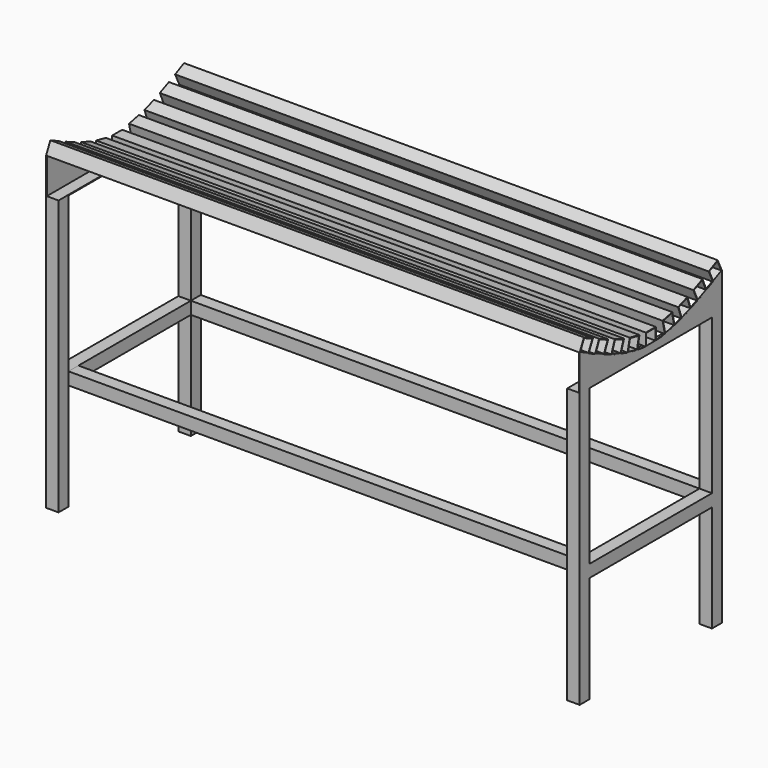
from build123d import *

# Parameters (mm, degrees)
F1_DEPTH  = 2
F2_W      = 35
F2_H      = 500
F3_DEPTH  = 2
F6_W      = 35
F6_H      = 35
F6_W_2    = 32
F6_H_2    = 32
F7_DEPTH  = 1500
F9_DEPTH  = 1500
F11_DEPTH = 1500
F13_DEPTH = 1500
F14_W     = 35
F14_H     = 35
F14_W_2   = 33
F14_H_2   = 33
F15_DEPTH = 770
F16_W     = 35
F16_H     = 35
F16_W_2   = 33
F16_H_2   = 33
F17_DEPTH = 770
F18_W     = 35
F18_H     = 35
F18_W_2   = 33
F18_H_2   = 33
F19_DEPTH = 440
F20_W     = 35
F20_H     = 35
F20_W_2   = 33
F20_H_2   = 33
F21_DEPTH = 440
F22_W     = 35
F22_H     = 35
F22_W_2   = 33
F22_H_2   = 33
F23_DEPTH = 1430
F24_W     = 35
F24_H     = 35
F24_W_2   = 33
F24_H_2   = 33
F25_DEPTH = 1430


with BuildPart() as f1:
    # F0 (on Right) → F1 (new body)
    with BuildSketch(Plane.YZ):
        with BuildLine():
            Line((-250, 50), (-250, -50))
            Line((-250, -50), (250, -50))
            Line((250, -50), (250, 50))
            add(Edge.make_bspline(
                [(250, 50), (166.6666666667, 10), (0, -70), (-166.6666666667, 10), (-250, 50)],
                knots=[0, 0, 0, 0, 0.5, 1, 1, 1, 1], degree=3))
        make_face()
    extrude(amount=F1_DEPTH)

    # F2 (on face) → F3 (join)
    with BuildSketch(Plane(origin=(0, 0, -50), x_dir=(1, 0, 0), z_dir=(0, 0, -1))):
        with Locations((17.5, 0)):
            Rectangle(F2_W, F2_H)
    extrude(amount=F3_DEPTH)


with BuildPart() as f4_1:
    # F4: instance of F1
    add(f1.part.mirror(Plane(origin=(35, 0, -51), x_dir=(0, 1, 0), z_dir=(1, 0, 0))))


with BuildPart() as f4_1_1:
    # F5: moved
    add(f4_1.part.moved(Location((1430, 0, 0))))

    # F16 (on face) → F17 (join)
    with BuildSketch(Plane(origin=(0, 0, -52), x_dir=(1, 0, 0), z_dir=(0, 0, -1))):
        with Locations((1482.5, 232.5)):
            Rectangle(F16_W, F16_H)
        with Locations((1482.5, 232.5)):
            Rectangle(F16_W_2, F16_H_2, mode=Mode.SUBTRACT)
        with Locations((1482.5, -232.5)):
            Rectangle(F16_W, F16_H)
        with Locations((1482.5, -232.5)):
            Rectangle(F16_W_2, F16_H_2, mode=Mode.SUBTRACT)
    extrude(amount=F17_DEPTH)

    # F18 (on face) → F19 (join)
    with BuildSketch(Plane.XZ.offset(-215)):
        with Locations((1482.5, -504.5)):
            Rectangle(F18_W, F18_H)
        with Locations((1482.5, -504.5)):
            Rectangle(F18_W_2, F18_H_2, mode=Mode.SUBTRACT)
    extrude(amount=F19_DEPTH)


with BuildPart() as f1_1:
    add(f1.part)

    # F6 (on face) → F7 (join)
    with BuildSketch(Plane(origin=(0, 0, 0), x_dir=(0, -1, 0), z_dir=(-1, 0, 0))):
        with Locations((0, -12.5)):
            Rectangle(F6_W, F6_H)
        with Locations((0, -12.5)):
            Rectangle(F6_W_2, F6_H_2, mode=Mode.SUBTRACT)
    extrude(amount=-F7_DEPTH)

    # F14 (on face) → F15 (join)
    with BuildSketch(Plane(origin=(0, 0, -52), x_dir=(1, 0, 0), z_dir=(0, 0, -1))):
        with Locations((17.5, 232.5)):
            Rectangle(F14_W, F14_H)
        with Locations((17.5, 232.5)):
            Rectangle(F14_W_2, F14_H_2, mode=Mode.SUBTRACT)
        with Locations((17.5, -232.5)):
            Rectangle(F14_W, F14_H)
        with Locations((17.5, -232.5)):
            Rectangle(F14_W_2, F14_H_2, mode=Mode.SUBTRACT)
    extrude(amount=F15_DEPTH)

    # F20 (on face) → F21 (join)
    with BuildSketch(Plane.XZ.offset(-215)):
        with Locations((17.5, -504.5)):
            Rectangle(F20_W, F20_H)
        with Locations((17.5, -504.5)):
            Rectangle(F20_W_2, F20_H_2, mode=Mode.SUBTRACT)
    extrude(amount=F21_DEPTH)


with BuildPart() as f9:
    # F8 (on face) → F9 (new body)
    with BuildSketch(Plane(origin=(0, 0, 0), x_dir=(0, -1, 0), z_dir=(-1, 0, 0))):
        Polygon((-234.9200030965, 81.5847066377), (-250, 50), (-218.4152933623, 34.9200030965), (-203.3352964588, 66.5047097342), align=None)
        Polygon((-234.2126583936, 79.5847907717), (-219.7739353592, 72.6910779015), (-205.3352123248, 65.7973650313), (-219.1226380652, 36.9199189626), (-248.0000841339, 50.7073447029), align=None, mode=Mode.SUBTRACT)
    extrude(amount=-F9_DEPTH)


with BuildPart() as f11:
    # F10 (on face) → F11 (new body)
    with BuildSketch(Plane(origin=(0, 0, 0), x_dir=(0, -1, 0), z_dir=(-1, 0, 0))):
        with BuildLine():
            add(Edge.make_bspline(
                [(-83.6444792813, -18.0650520534), (-72.2522280284, -21.1120515617), (-60.8599767755, -23.6616132493), (-49.4677255225, -25.6115414701)],
                knots=[0.3327110414, 0.3327110414, 0.3327110414, 0.3327110414, 0.401064549, 0.401064549, 0.401064549, 0.401064549], degree=3))
            Line((-49.4677255225, -25.6115414701), (-41.5525741961, 10.2348187258))
            Line((-41.5525741961, 10.2348187258), (-75.7293279548, 17.7813081425))
            Line((-75.7293279548, 17.7813081425), (-83.6444792813, -18.0650520534))
        make_face()
        Polygon((-74.6562526953, 16.0082330425), (-58.9643720505, 12.5433454159), (-43.2724914057, 9.0784577893), (-50.5408007821, -23.8384663701), (-81.9245620717, -16.9086911169), align=None, mode=Mode.SUBTRACT)
    extrude(amount=-F11_DEPTH)


with BuildPart() as f11b:
    # F10 (on face) → F11, piece 2 (new body)
    with BuildSketch(Plane(origin=(0, 0, 0), x_dir=(0, -1, 0), z_dir=(-1, 0, 0))):
        Polygon((-140.569047312, 0.8278953682), (-107.6123605236, -10.955855984), (-95.8286091714, 22.0008308044), (-128.7852959598, 33.7845821566), align=None)
        Polygon((-127.8778844411, 31.8671348077), (-112.8119704807, 26.4802770467), (-97.7460565203, 21.0934192857), (-108.5197720423, -9.0384086351), (-138.6515999631, 1.7353068869), align=None, mode=Mode.SUBTRACT)
    extrude(amount=-F11_DEPTH)


with BuildPart() as f11c:
    # F10 (on face) → F11, piece 3 (new body)
    with BuildSketch(Plane(origin=(0, 0, 0), x_dir=(0, -1, 0), z_dir=(-1, 0, 0))):
        Polygon((-195.7508154323, 24.3691054968), (-163.7317283517, 10.2348187258), (-149.5974415807, 42.2539058064), (-181.6165286613, 56.3881925774), align=None)
        Polygon((-180.8503805606, 54.4110768645), (-166.1714005224, 47.9312883295), (-151.5745572935, 41.4877577057), (-164.4978764523, 12.2119344387), (-193.7736997194, 25.1352535974), align=None, mode=Mode.SUBTRACT)
    extrude(amount=-F11_DEPTH)


with BuildPart() as f13:
    # F12 (on face) → F13 (new body)
    with BuildSketch(Plane(origin=(0, 0, 0), x_dir=(0, -1, 0), z_dir=(-1, 0, 0))):
        Polygon((218.4152933623, 34.9200030965), (250, 50), (234.9200030965, 81.5847066377), (203.3352964588, 66.5047097342), align=None)
        Polygon((205.3352123248, 65.7973650313), (219.7739353592, 72.6910779015), (234.2126583936, 79.5847907717), (248.0000841339, 50.7073447029), (219.1226380652, 36.9199189626), align=None, mode=Mode.SUBTRACT)
    extrude(amount=-F13_DEPTH)


with BuildPart() as f13b:
    # F12 (on face) → F13, piece 2 (new body)
    with BuildSketch(Plane(origin=(0, 0, 0), x_dir=(0, -1, 0), z_dir=(-1, 0, 0))):
        Polygon((163.7317283517, 10.2348187258), (195.7508154323, 24.3691054968), (181.6165286613, 56.3881925774), (149.5974415807, 42.2539058064), align=None)
        Polygon((151.5754433172, 41.4874143645), (166.2127402683, 47.9488026027), (180.8500372194, 54.4101908409), (193.7728136958, 25.1355969386), (164.4982197935, 12.2128204623), align=None, mode=Mode.SUBTRACT)
    extrude(amount=-F13_DEPTH)


with BuildPart() as f13c:
    # F12 (on face) → F13, piece 3 (new body)
    with BuildSketch(Plane(origin=(0, 0, 0), x_dir=(0, -1, 0), z_dir=(-1, 0, 0))):
        Polygon((105.4247818059, -11.6600143596), (138.4254494527, 0), (126.7654350931, 33.0006676468), (93.7647674463, 21.3406532872), align=None)
        Polygon((95.6787966751, 20.4260538606), (110.7648161708, 25.7563461393), (125.8508356665, 31.0866384179), (136.5114202239, 0.9145994266), (106.3393812325, -9.7459851308), align=None, mode=Mode.SUBTRACT)
    extrude(amount=-F13_DEPTH)


with BuildPart() as f13d:
    # F12 (on face) → F13, piece 4 (new body)
    with BuildSketch(Plane(origin=(0, 0, 0), x_dir=(0, -1, 0), z_dir=(-1, 0, 0))):
        Polygon((47.200742599, -25.9916196732), (81.4227235681, -18.6529536807), (74.0840575757, 15.5690272884), (39.8620766065, 8.230361296), align=None)
        Polygon((41.6432471906, 7.0782192255), (57.2875813479, 10.4330379649), (72.9319155052, 13.7878567043), (79.641552984, -17.5008116103), (48.3528846694, -24.2104490891), align=None, mode=Mode.SUBTRACT)
    extrude(amount=-F13_DEPTH)


with BuildPart() as f23:
    # F22 (on face) → F23 (new body)
    with BuildSketch(Plane.YZ.offset(35)):
        with Locations((232.5, -504.5)):
            Rectangle(F22_W, F22_H)
        with Locations((232.5, -504.5)):
            Rectangle(F22_W_2, F22_H_2, mode=Mode.SUBTRACT)
    extrude(amount=F23_DEPTH)


with BuildPart() as f25:
    # F24 (on face) → F25 (new body)
    with BuildSketch(Plane.YZ.offset(35)):
        with Locations((-197.5, -504.5)):
            Rectangle(F24_W, F24_H)
        with Locations((-197.5, -504.5)):
            Rectangle(F24_W_2, F24_H_2, mode=Mode.SUBTRACT)
    extrude(amount=F25_DEPTH)


solid = Compound([f4_1_1.part, f1_1.part, f9.part, f11.part, f11b.part, f11c.part, f13.part, f13b.part, f13c.part, f13d.part, f23.part, f25.part])
